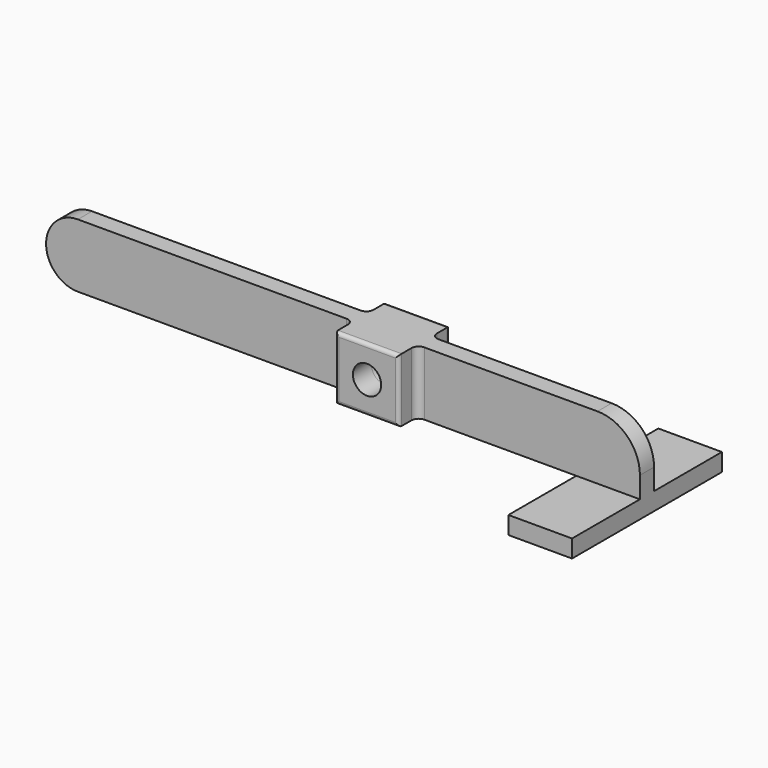
from build123d import *

# Parameters (mm, degrees)
F1_DEPTH = 57.15
F2_R     = 3.175
F3_R     = 28.57499
F5_D     = 25.4
F5_DEPTH = 38.1
F5_TIP   = 7.6309298617
F6_D     = 25.4
F7_R     = 38.1
F9_DEPTH = 15.875


# Not quite as in the source:
# - a fillet or chamfer is up to 0.001 mm smaller than in the source, because OpenCascade refuses the exact size
# - a length typed as a fraction of an inch, garbled in the dataset ("3 / 203.2 mm" for 3/8 in), is restored


with BuildPart() as f1:
    # F0 (on Top) → F1 (new body)
    with BuildSketch(Plane.XY):
        with BuildLine():
            ThreePointArc((28.575, -6.35), (30.4348719395, -1.8598719395), (34.925, 0))
            Line((34.925, 0), (228.6, 0))
            Line((228.6, 0), (228.6, 15.875))
            Line((228.6, 15.875), (34.925, 15.875))
            ThreePointArc((34.925, 15.875), (30.4348719395, 17.7348719395), (28.575, 22.225))
            Line((28.575, 22.225), (28.575, 36.5125))
            Line((28.575, 36.5125), (0, 36.5125))
            Line((0, 36.5125), (-28.575, 36.5125))
            Line((-28.575, 36.5125), (-28.575, 22.225))
            ThreePointArc((-28.575, 22.225), (-30.4348719395, 17.7348719395), (-34.925, 15.875))
            Line((-34.925, 15.875), (-304.8, 15.875))
            Line((-304.8, 15.875), (-304.8, 0))
            Line((-304.8, 0), (-34.925, 0))
            ThreePointArc((-34.925, 0), (-30.4348719395, -1.8598719395), (-28.575, -6.35))
            Line((-28.575, -6.35), (-28.575, -20.6375))
            Line((-28.575, -20.6375), (0, -20.6375))
            Line((0, -20.6375), (28.575, -20.6375))
            Line((28.575, -20.6375), (28.575, -6.35))
        make_face()
    extrude(amount=F1_DEPTH)

    # F2
    f2_edges = [f1.edges().sort_by_distance(p)[0] for p in [
        (28.575, 36.5125, 28.575),
        (0, 36.5125, 57.15),
        (-28.575, 36.5125, 28.575),
        (0, 36.5125, 0),
        (-28.575, -20.6375, 28.575),
        (0, -20.6375, 57.15),
        (28.575, -20.6375, 28.575),
        (0, -20.6375, 0),
    ]]
    fillet(f2_edges, radius=F2_R)

    # F3 (radius 28.575 in the source; OpenCascade refuses exactly that, so slightly less here)
    f3_edges = [f1.edges().sort_by_distance(p)[0] for p in [
        (-304.8, 7.9375, 57.15),
        (-304.8, 7.9375, 0),
    ]]
    fillet(f3_edges, radius=F3_R)

    # F5 (one way)
    with BuildSketch(Plane.XZ):
        with Locations((0, 28.575)):
            Circle(F5_D / 2)
    extrude(amount=-F5_DEPTH, mode=Mode.SUBTRACT)
    with Locations(Plane.XZ):
        with Locations((0, 28.575)):
            with Locations((0, 0, -(F5_DEPTH + F5_TIP / 2))):  # 118° drill point
                Cone(0, F5_D / 2, F5_TIP, mode=Mode.SUBTRACT)

    # F6 (through all)
    with Locations(Plane(origin=(0, 0, 0), x_dir=(1, 0, 0), z_dir=(0, 1, 0))):
        with Locations((0, -28.575)):
            Hole(F6_D / 2)

    # F7
    f7_edges = [f1.edges().sort_by_distance(p)[0] for p in [
        (228.6, 7.9375, 57.15),
    ]]
    fillet(f7_edges, radius=F7_R)

    # F8 (on Top) → F9 (join)
    with BuildSketch(Plane.XY):
        Polygon((228.6, -76.2), (228.6, 0), (228.6, 92.075), (171.45, 92.075), (171.45, -76.2), align=None)
    extrude(amount=-F9_DEPTH)


solid = f1.part
